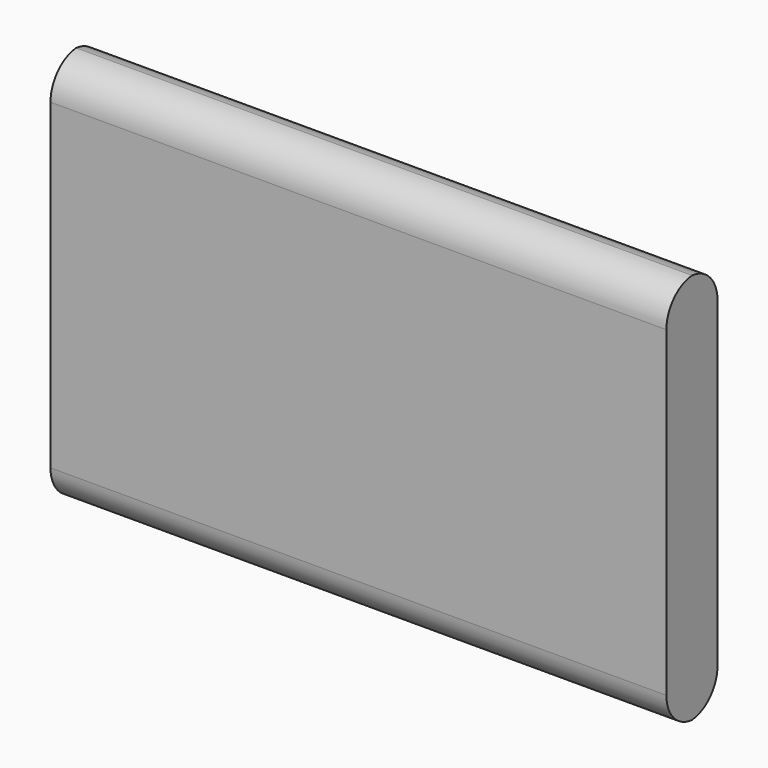
from build123d import *

# Parameters (mm, degrees)
F0_W        = 53
F0_H        = 33.7
F1_DEPTH    = 5.5
F2_T1_DEPTH = 68


# Not quite as in the source:
# - a fillet or chamfer that OpenCascade refuses, or shapes differently, is made with other operations: its cross-section is extruded or revolved along the edge and cut away or added


with BuildPart() as f1:
    # F0 (on Front) → F1 (new body)
    with BuildSketch(Plane.XZ):
        with Locations((-24.1282908246, 38.41047619)):
            Rectangle(F0_W, F0_H)
    extrude(amount=F1_DEPTH)

    # F2: fillet of radius 3 on 4 edges, made by hand

    # F2_s2 → F2_t1 (cut)
    with BuildSketch(Plane.YZ.offset(-58.1282908246)):
        with BuildLine():
            ThreePointArc((-2.5, 55.26047619), (-4.6213203436, 54.3817965336), (-5.5, 52.26047619))
            Line((-5.5, 52.26047619), (-5.5, 55.26047619))
            Line((-5.5, 55.26047619), (-2.5, 55.26047619))
        make_face()
        with BuildLine():
            ThreePointArc((-3, 55.26047619), (-0.8786796564, 54.3817965336), (0, 52.26047619))
            Line((0, 52.26047619), (0, 55.26047619))
            Line((0, 55.26047619), (-3, 55.26047619))
        make_face()
        with BuildLine():
            ThreePointArc((-3, 21.56047619), (-0.8786796564, 22.4391558465), (0, 24.56047619))
            Line((0, 24.56047619), (0, 21.56047619))
            Line((0, 21.56047619), (-3, 21.56047619))
        make_face()
        with BuildLine():
            ThreePointArc((-2.5, 21.56047619), (-4.6213203436, 22.4391558465), (-5.5, 24.56047619))
            Line((-5.5, 24.56047619), (-5.5, 21.56047619))
            Line((-5.5, 21.56047619), (-2.5, 21.56047619))
        make_face()
    extrude(amount=F2_T1_DEPTH, mode=Mode.SUBTRACT)


solid = f1.part
